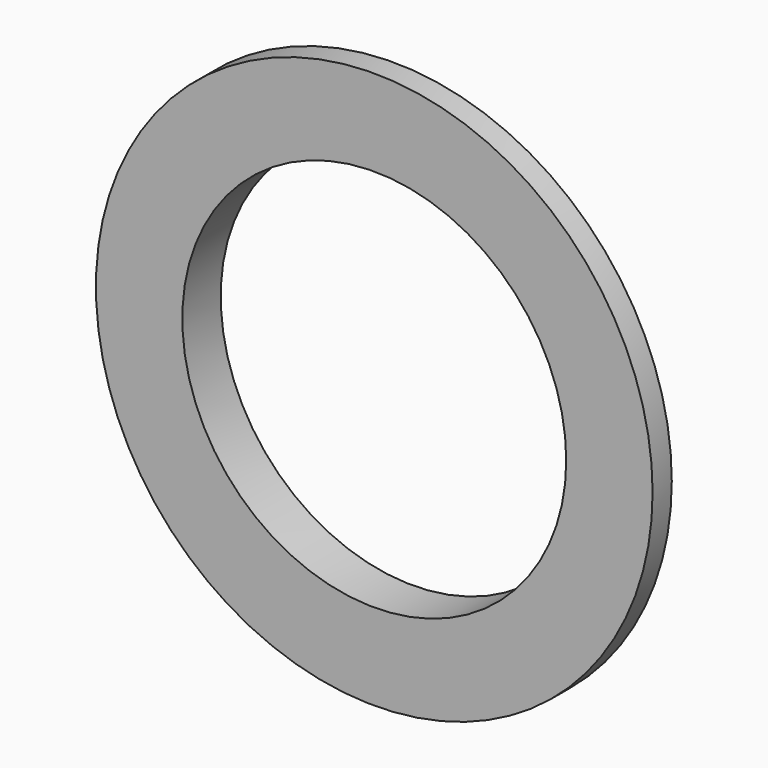
from build123d import *

# Parameters (mm, degrees)
F0_R     = 29
F0_R_2   = 25
F0_R_3   = 23
F0_R_4   = 20
F1_DEPTH = 2.5
F2_DEPTH = 2.5


# Not quite as in the source:
# - the program builds the solid bodies; features that only make, move or delete a surface that nothing else refers to are left out


with BuildPart() as f1:
    # F0 (on Front) → F1 (new body)
    with BuildSketch(Plane.XZ):
        Circle(F0_R)
        Circle(F0_R_2, mode=Mode.SUBTRACT)
        Circle(F0_R_2)
        Circle(F0_R_3, mode=Mode.SUBTRACT)
        Circle(F0_R_3)
        Circle(F0_R_4, mode=Mode.SUBTRACT)
    extrude(amount=F1_DEPTH)

    # F0 (on Front) → F2 (join, symmetric)
    with BuildSketch(Plane.XZ):
        Circle(F0_R_2)
        Circle(F0_R_3, mode=Mode.SUBTRACT)
        Circle(F0_R_3)
        Circle(F0_R_4, mode=Mode.SUBTRACT)
    extrude(amount=F2_DEPTH, both=True)


solid = f1.part
